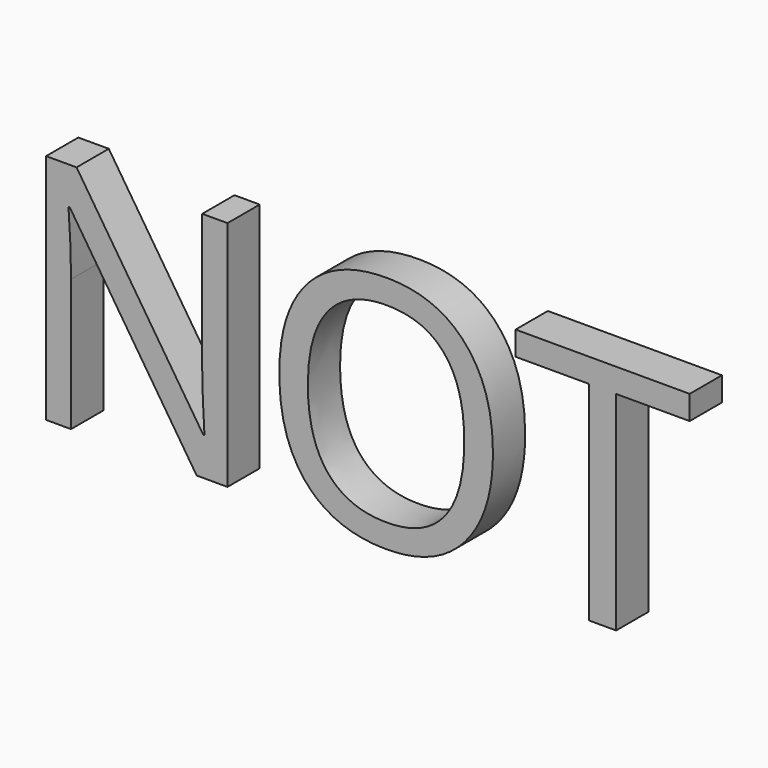
from build123d import *

# Parameters (mm, degrees)
F0_TEXT_SIZE = 80.7455068247
F1_DEPTH     = 10


# Not quite as in the source:
# - Text() gives the source's letters only with a copy of the font that has no kerning and outlines rounded to 1/6400 em; it was checked with that copy


with BuildPart() as f1:
    # F0 (on Front) → F1 (new body)
    with BuildSketch(Plane.XZ):
        with Locations((-43.8903793693, -26.0464213789)):
            Text('NOT', F0_TEXT_SIZE, font='Open Sans', text_align=(TextAlign.LEFT, TextAlign.BOTTOM))
    extrude(amount=F1_DEPTH)


solid = f1.part
